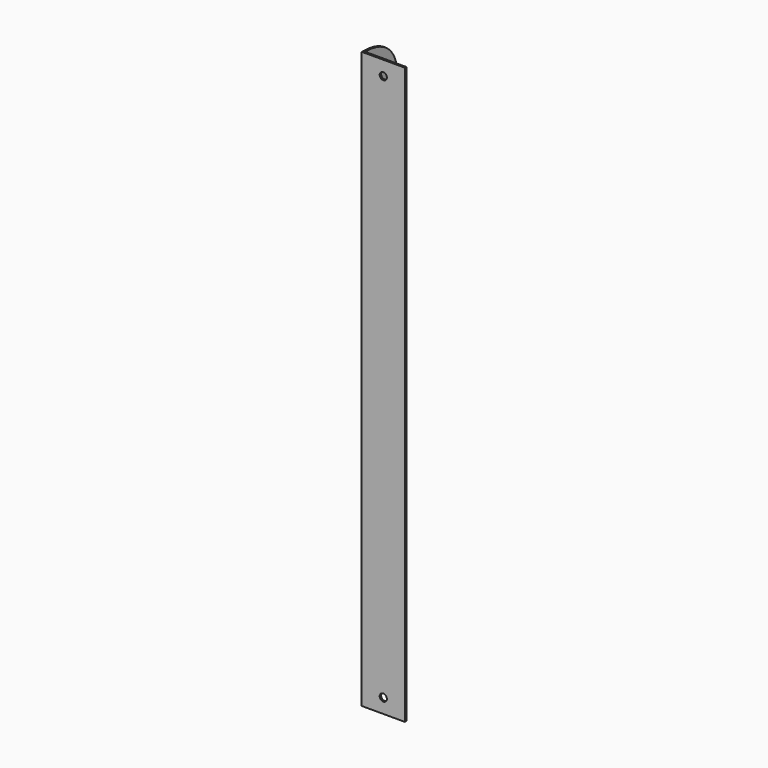
from build123d import *

# Parameters (mm, degrees)
F1_DEPTH    = 508
F2_T1_DEPTH = 192.0875
F3_R        = 3.175
F4_DEPTH    = 1.5875
F5_R        = 3.175
F6_DEPTH    = 1.5875


# Not quite as in the source:
# - a fillet or chamfer that OpenCascade refuses, or shapes differently, is made with other operations: its cross-section is extruded or revolved along the edge and cut away or added


with BuildPart() as f1:
    # F0 (on Top) → F1 (new body)
    with BuildSketch(Plane.XY):
        Polygon((-11.3587090754, 18.7056229889), (-12.9462090754, 18.7056229889), (-12.9462090754, -19.3943770111), (25.1537909246, -19.3943770111), (25.1537909246, -17.8068770111), (-11.3587090754, -17.8068770111), align=None)
    extrude(amount=F1_DEPTH)

    # F2: fillet of radius 38.1 on 2 edges, made by hand

    # F2_s2 → F2_t1 (cut)
    with BuildSketch(Plane.YZ.offset(-108.1962090754)):
        with BuildLine():
            add(Edge.make_bspline(
                [(18.7056229889, 469.9), (18.7056229889, 508), (-19.3943770111, 508)],
                knots=[0, 0, 0, 1, 1, 1], degree=2, weights=[1, 1, 1]))
            Line((-19.3943770111, 508), (18.7056229889, 508))
            Line((18.7056229889, 508), (18.7056229889, 469.9))
        make_face()
        with BuildLine():
            add(Edge.make_bspline(
                [(18.7056229889, 38.1), (18.7056229889, 0), (-19.3943770111, 0)],
                knots=[0, 0, 0, 1, 1, 1], degree=2, weights=[1, 1, 1]))
            Line((-19.3943770111, 0), (18.7056229889, 0))
            Line((18.7056229889, 0), (18.7056229889, 38.1))
        make_face()
    extrude(amount=F2_T1_DEPTH, mode=Mode.SUBTRACT)

    # F3 (on face) → F4 (cut)
    with BuildSketch(Plane(origin=(-12.9462090754, 0, 0), x_dir=(0, -1, 0), z_dir=(-1, 0, 0))):
        with Locations((0.3443770111, 488.9331097904)):
            Circle(F3_R)
        with Locations((0.3443770111, 19.0668902096)):
            Circle(F3_R)
    extrude(amount=-F4_DEPTH, mode=Mode.SUBTRACT)

    # F5 (on face) → F6 (cut)
    with BuildSketch(Plane.XZ.offset(19.3943770111)):
        with Locations((6.1037909246, 12.7)):
            Circle(F5_R)
        with Locations((6.1037909246, 495.3)):
            Circle(F5_R)
    extrude(amount=-F6_DEPTH, mode=Mode.SUBTRACT)


solid = f1.part
